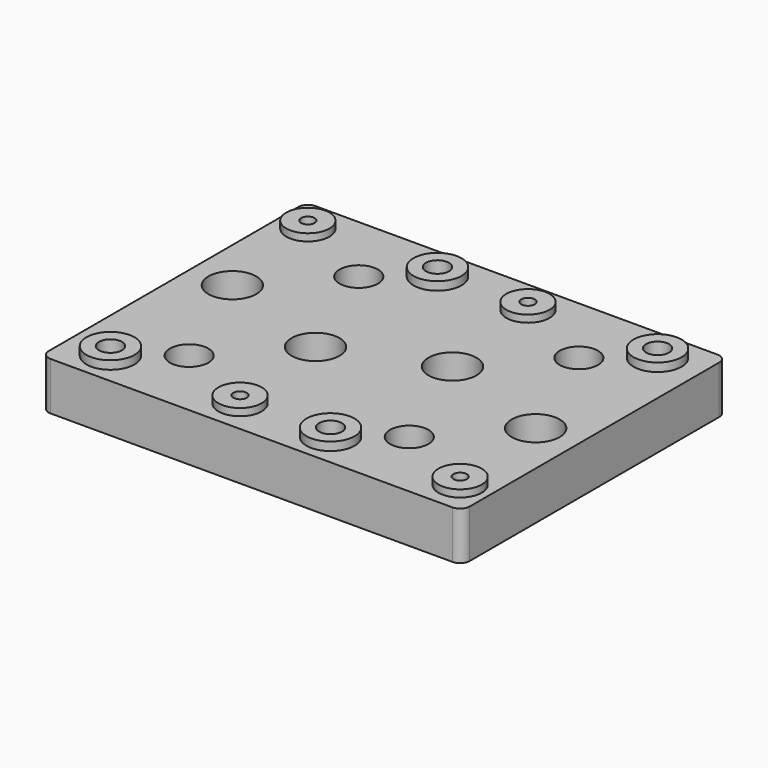
from build123d import *

# Parameters (mm, degrees)
F0_W         = 87.7034852714
F0_H         = 68.9755799484
F0_R         = 2.395
F0_R_2       = 4
F0_R_3       = 1.405
F0_R_4       = 5
F1_DEPTH     = 10
F2_R         = 2
F3_R         = 4.5
F3_R_2       = 1.405
F4_DEPTH     = 1.5
F5_TEXT_SIZE = 7.964369924
F6_DEPTH     = 1
F3_R_3       = 5
F3_R_4       = 2.395
F7_DEPTH     = 1.75


# Not quite as in the source:
# - Text() gives the source's letters only with a copy of the font that has no kerning and outlines rounded to 1/6400 em; it was checked with that copy


with BuildPart() as f1:
    # F0 (on Top) → F1 (new body)
    with BuildSketch(Plane.XY):
        with Locations((0, 34.4877899742)):
            Rectangle(F0_W, F0_H)
        with Locations((-35, 7)):
            Circle(F0_R, mode=Mode.SUBTRACT)
        with Locations((-25, 15)):
            Circle(F0_R_2, mode=Mode.SUBTRACT)
        with Locations((-8, 7)):
            Circle(F0_R_3, mode=Mode.SUBTRACT)
        with Locations((-10.8517426357, 30.2255799484)):
            Circle(F0_R_4, mode=Mode.SUBTRACT)
        with Locations((10.8517426357, 7)):
            Circle(F0_R, mode=Mode.SUBTRACT)
        with Locations((20.8517426357, 15)):
            Circle(F0_R_2, mode=Mode.SUBTRACT)
        with Locations((37.8517426357, 7)):
            Circle(F0_R_3, mode=Mode.SUBTRACT)
        with Locations((35, 30.2255799484)):
            Circle(F0_R_4, mode=Mode.SUBTRACT)
        with Locations((-35, 38.75)):
            Circle(F0_R_4, mode=Mode.SUBTRACT)
        with Locations((-37.8517426357, 61.9755799484)):
            Circle(F0_R_3, mode=Mode.SUBTRACT)
        with Locations((-20.8517426357, 53.9755799484)):
            Circle(F0_R_2, mode=Mode.SUBTRACT)
        with Locations((-10.8517426357, 61.9755799484)):
            Circle(F0_R, mode=Mode.SUBTRACT)
        with Locations((10.8517426357, 38.75)):
            Circle(F0_R_4, mode=Mode.SUBTRACT)
        with Locations((8, 61.9755799484)):
            Circle(F0_R_3, mode=Mode.SUBTRACT)
        with Locations((25, 53.9755799484)):
            Circle(F0_R_2, mode=Mode.SUBTRACT)
        with Locations((35, 61.9755799484)):
            Circle(F0_R, mode=Mode.SUBTRACT)
    extrude(amount=F1_DEPTH)

    # F2
    f2_edges = [f1.edges().sort_by_distance(p)[0] for p in [
        (-43.851743, 0, 5),
        (43.851743, 0, 5),
        (43.851743, 68.97558, 5),
        (-43.851743, 68.97558, 5),
    ]]
    fillet(f2_edges, radius=F2_R)

    # F3 (on face) → F4 (join)
    with BuildSketch(Plane.XY.offset(10)):
        with Locations((-37.8517426357, 61.9755799484)):
            Circle(F3_R)
        with Locations((-37.8517426357, 61.9755799484)):
            Circle(F3_R_2, mode=Mode.SUBTRACT)
        with Locations((8, 61.9755799484)):
            Circle(F3_R)
        with Locations((8, 61.9755799484)):
            Circle(F3_R_2, mode=Mode.SUBTRACT)
        with Locations((37.8517426357, 7)):
            Circle(F3_R)
        with Locations((37.8517426357, 7)):
            Circle(F3_R_2, mode=Mode.SUBTRACT)
        with Locations((-8, 7)):
            Circle(F3_R)
        with Locations((-8, 7)):
            Circle(F3_R_2, mode=Mode.SUBTRACT)
    extrude(amount=F4_DEPTH)

    # F5 (on face) → F6 (cut)
    with BuildSketch(Plane(origin=(-43.8517426357, 0, 0), x_dir=(0, -1, 0), z_dir=(-1, 0, 0))):
        with Locations((-44, 2.6328268274)):
            Text('O-043-001', F5_TEXT_SIZE, font='Open Sans', font_style=FontStyle.BOLD, text_align=(TextAlign.LEFT, TextAlign.BOTTOM))
    extrude(amount=-F6_DEPTH, mode=Mode.SUBTRACT)

    # F3 (on face) → F7 (join)
    with BuildSketch(Plane.XY.offset(10)):
        with Locations((-10.8517426357, 61.9755799484)):
            Circle(F3_R_3)
        with Locations((-10.8517426357, 61.9755799484)):
            Circle(F3_R_4, mode=Mode.SUBTRACT)
        with Locations((-35, 7)):
            Circle(F3_R_3)
        with Locations((-35, 7)):
            Circle(F3_R_4, mode=Mode.SUBTRACT)
        with Locations((35, 61.9755799484)):
            Circle(F3_R_3)
        with Locations((35, 61.9755799484)):
            Circle(F3_R_4, mode=Mode.SUBTRACT)
        with Locations((10.8517426357, 7)):
            Circle(F3_R_3)
        with Locations((10.8517426357, 7)):
            Circle(F3_R_4, mode=Mode.SUBTRACT)
    extrude(amount=F7_DEPTH)


solid = f1.part
